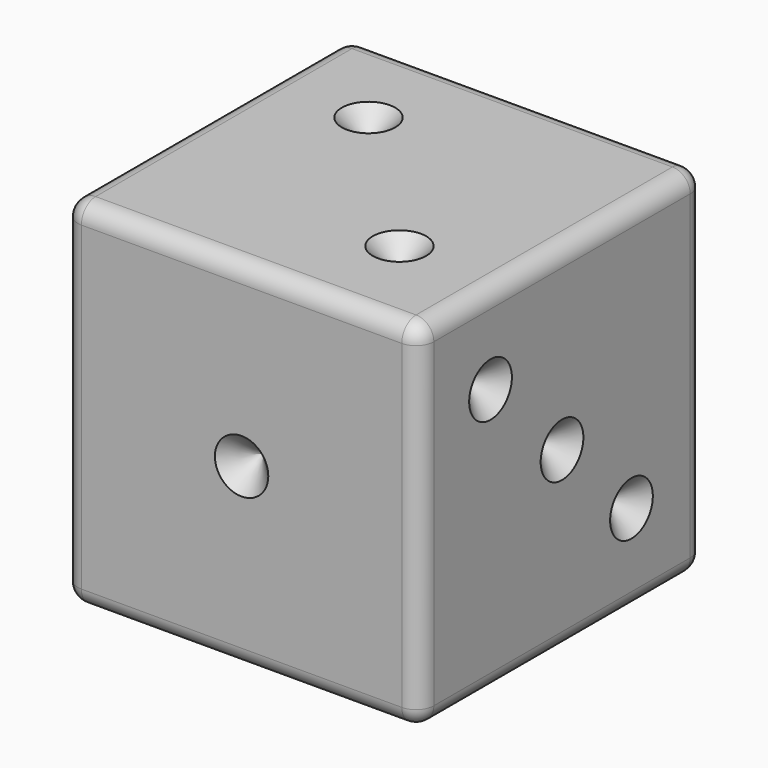
from build123d import *

# Parameters (mm, degrees)
F0_W      = 20
F0_H      = 20
F1_DEPTH  = 20
F2_R      = 1.5
F3_DEPTH  = 1.5
F4_R      = 1
F5_SIZE   = 1.49999
F9_R      = 1.5
F10_DEPTH = 1.5
F11_SIZE  = 1.49999
F8_R      = 1.5
F12_DEPTH = 1.5
F13_SIZE  = 1.49999
F6_R      = 1.5
F14_DEPTH = 1.5
F15_SIZE  = 1.49999
F7_R      = 1.5
F16_DEPTH = 1.5
F17_SIZE  = 1.49999
F18_R     = 1.5
F19_DEPTH = 1.5
F20_SIZE  = 1.49999


# Not quite as in the source:
# - a fillet or chamfer is up to 0.001 mm smaller than in the source, because OpenCascade refuses the exact size


with BuildPart() as f1:
    # F0 (on Top) → F1 (new body)
    with BuildSketch(Plane.XY):
        with Locations((10, 10)):
            Rectangle(F0_W, F0_H)
    extrude(amount=F1_DEPTH)

    # F2 (on face) → F3 (cut)
    with BuildSketch(Plane.XZ):
        with Locations((10, 10)):
            Circle(F2_R)
    extrude(amount=-F3_DEPTH, mode=Mode.SUBTRACT)

    # F4
    f4_edges = [f1.edges().sort_by_distance(p)[0] for p in [
        (0, 10, 20),
        (20, 10, 20),
        (20, 10, 0),
        (0, 10, 0),
        (0, 0, 10),
        (20, 0, 10),
        (20, 20, 10),
        (10, 20, 20),
        (0, 20, 10),
        (10, 0, 0),
        (10, 20, 0),
        (10, 0, 20),
    ]]
    fillet(f4_edges, radius=F4_R)

    # F5 (size 1.5 in the source; OpenCascade refuses exactly that, so slightly less here)
    f5_edges = [f1.edges().sort_by_distance(p)[0] for p in [
        (8.5, 1.5, 10),
    ]]
    chamfer(f5_edges, length=F5_SIZE)

    # F9 (on face) → F10 (cut)
    with BuildSketch(Plane(origin=(0, 0, 0), x_dir=(0, -1, 0), z_dir=(-1, 0, 0))):
        with Locations((-5.6568542495, 14.3431457505)):
            Circle(F9_R)
        with Locations((-10, 10)):
            Circle(F9_R)
        with Locations((-14.3431457505, 5.6568542495)):
            Circle(F9_R)
        with Locations((-5.6568542495, 5.6568542495)):
            Circle(F9_R)
        with Locations((-14.3431457505, 14.3431457505)):
            Circle(F9_R)
    extrude(amount=-F10_DEPTH, mode=Mode.SUBTRACT)

    # F11 (size 1.5 in the source; OpenCascade refuses exactly that, so slightly less here)
    f11_edges = [f1.edges().sort_by_distance(p)[0] for p in [
        (1.5, 11.5, 10),
        (1.5, 15.843146, 5.656854),
        (1.5, 15.843146, 14.343146),
        (1.5, 7.156854, 14.343146),
        (1.5, 7.156854, 5.656854),
    ]]
    chamfer(f11_edges, length=F11_SIZE)

    # F8 (on face) → F12 (cut)
    with BuildSketch(Plane(origin=(0, 0, 0), x_dir=(1, 0, 0), z_dir=(0, 0, -1))):
        with Locations((6.9175572135, -5)):
            Circle(F8_R)
        with Locations((13.4148458019, -5)):
            Circle(F8_R)
        with Locations((6.9175572135, -10)):
            Circle(F8_R)
        with Locations((13.4148458019, -10)):
            Circle(F8_R)
        with Locations((6.9175572135, -15)):
            Circle(F8_R)
        with Locations((13.4148458019, -15)):
            Circle(F8_R)
    extrude(amount=-F12_DEPTH, mode=Mode.SUBTRACT)

    # F13 (size 1.5 in the source; OpenCascade refuses exactly that, so slightly less here)
    f13_edges = [f1.edges().sort_by_distance(p)[0] for p in [
        (5.417557, 5, 1.5),
        (11.914846, 5, 1.5),
        (5.417557, 10, 1.5),
        (11.914846, 10, 1.5),
        (11.914846, 15, 1.5),
        (5.417557, 15, 1.5),
    ]]
    chamfer(f13_edges, length=F13_SIZE)

    # F6 (on face) → F14 (cut)
    with BuildSketch(Plane.YZ.offset(20)):
        with Locations((4.979637754, 15.020362246)):
            Circle(F6_R)
        with Locations((10.0000959005, 9.9999040995)):
            Circle(F6_R)
        with Locations((14.8777184771, 5.1222815229)):
            Circle(F6_R)
    extrude(amount=-F14_DEPTH, mode=Mode.SUBTRACT)

    # F15 (size 1.5 in the source; OpenCascade refuses exactly that, so slightly less here)
    f15_edges = [f1.edges().sort_by_distance(p)[0] for p in [
        (18.5, 3.479638, 15.020362),
        (18.5, 8.500096, 9.999904),
        (18.5, 13.377718, 5.122282),
    ]]
    chamfer(f15_edges, length=F15_SIZE)

    # F7 (on face) → F16 (cut)
    with BuildSketch(Plane(origin=(0, 20, 0), x_dir=(-1, 0, 0), z_dir=(0, 1, 0))):
        with Locations((-14.3431457505, 14.3431457505)):
            Circle(F7_R)
        with Locations((-5.6568542495, 14.3431457505)):
            Circle(F7_R)
        with Locations((-14.3431457505, 5.6568542495)):
            Circle(F7_R)
        with Locations((-5.6568542495, 5.6568542495)):
            Circle(F7_R)
    extrude(amount=-F16_DEPTH, mode=Mode.SUBTRACT)

    # F17 (size 1.5 in the source; OpenCascade refuses exactly that, so slightly less here)
    f17_edges = [f1.edges().sort_by_distance(p)[0] for p in [
        (15.843146, 18.5, 14.343146),
        (7.156854, 18.5, 14.343146),
        (7.156854, 18.5, 5.656854),
        (15.843146, 18.5, 5.656854),
    ]]
    chamfer(f17_edges, length=F17_SIZE)

    # F18 (on face) → F19 (cut)
    with BuildSketch(Plane.XY.offset(20)):
        with Locations((5.6568542495, 14.3431457505)):
            Circle(F18_R)
        with Locations((14.3431457505, 5.6568542495)):
            Circle(F18_R)
    extrude(amount=-F19_DEPTH, mode=Mode.SUBTRACT)

    # F20 (size 1.5 in the source; OpenCascade refuses exactly that, so slightly less here)
    f20_edges = [f1.edges().sort_by_distance(p)[0] for p in [
        (4.156854, 14.343146, 18.5),
        (12.843146, 5.656854, 18.5),
    ]]
    chamfer(f20_edges, length=F20_SIZE)


solid = f1.part
